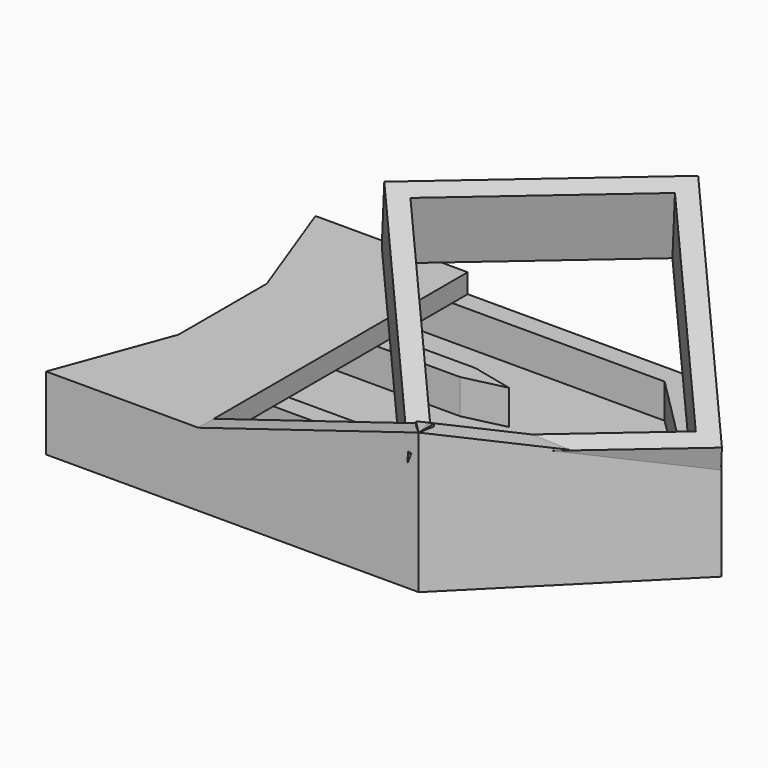
from build123d import *

# Parameters (mm, degrees)
F1_DEPTH  = 1.4
F3_DEPTH  = 2.5
F5_DEPTH  = 1.4
F7_DEPTH  = 1.4
F9_DEPTH  = 1.4
F14_DEPTH = 5


with BuildPart() as f1:
    # F0 (on Top) → F1 (new body)
    with BuildSketch(Plane.XY):
        Polygon((27, 12.2), (0, 12.2), (3.0312324917, 4), (3.0312324917, 0), (3.0312324917, -4), (0, -12.2), (27, -12.2), (39.2, 0), align=None)
    extrude(amount=F1_DEPTH)

    # F2 (on face) → F3 (join)
    with BuildSketch(Plane.XY.offset(1.4)):
        Polygon((3.0312324917, -4), (2.5137049932, -5.4), (17.0312324917, -5.4), (20.0312324917, -4.7), (17.0312324917, -4), align=None)
        Polygon((17.0312324917, 5.4), (2.5137049932, 5.4), (3.0312324917, 4), (17.0312324917, 4), (20.0312324917, 4.7), align=None)
        Polygon((0.5175274986, -10.8), (0, -12.2), (27, -12.2), (39.2, 0), (27, 12.2), (0, 12.2), (0.5175274986, 10.8), (26.4201010127, 10.8), (37.2201010127, 0), (26.4201010127, -10.8), align=None)
    extrude(amount=F3_DEPTH)

    # F4 (on face) → F5 (join)
    with BuildSketch(Plane.XY.offset(3.9)):
        Polygon((11.0312324917, 12.2), (0, 12.2), (2.5137049932, 5.4), (3.0312324917, 4), (3.0312324917, -4), (11.0312324917, -4), align=None)
        Polygon((11.0312324917, -5.4), (11.0312324917, -4), (3.0312324917, -4), (2.5137049932, -5.4), align=None)
        Polygon((11.0312324917, -12.2), (11.0312324917, -5.4), (2.5137049932, -5.4), (0, -12.2), align=None)
    extrude(amount=F5_DEPTH)

    # F6 (on face) → F7 (join, through all)
    with BuildSketch(Plane.XZ.offset(12.2)):
        Polygon((27, 10.1821421724), (11.0312324917, 5.3), (11.0312324917, 3.9), (27, 3.9), align=None)
    extrude(amount=-F7_DEPTH)

    # F8 (on face) → F9 (join)
    with BuildSketch(Plane(origin=(19.6, -19.6, 0), x_dir=(0.7071067812, 0.7071067812, 0), z_dir=(0.7071067812, -0.7071067812, 0))):
        Polygon((27.7185858225, 6.9844124824), (10.4651803616, 10.1821421724), (10.4651803616, 3.9), (27.7185858225, 3.9), align=None)
    extrude(amount=-F9_DEPTH)

    # F13 (on face) → F14 (join)
    with BuildSketch(Plane(origin=(2.8302744437, -2.8302744437, 14.9379532259), x_dir=(0.9831105487, 0.0340690567, -0.1798136492), z_dir=(-0.1830127019, 0.1830127019, -0.9659258263))):
        Polygon((8.8699151639, -6.6390948271), (22.2504726779, -18.3779482896), (37.2867568883, -1.2388072043), (23.9061993743, 10.5000462583), align=None)
        Polygon((10.8455991733, -6.5099720365), (24.0353221649, 8.5243622489), (35.3110728789, -1.3679299948), (22.1213498873, -16.4022642802), align=None, mode=Mode.SUBTRACT)
    extrude(amount=F14_DEPTH)


solid = f1.part
